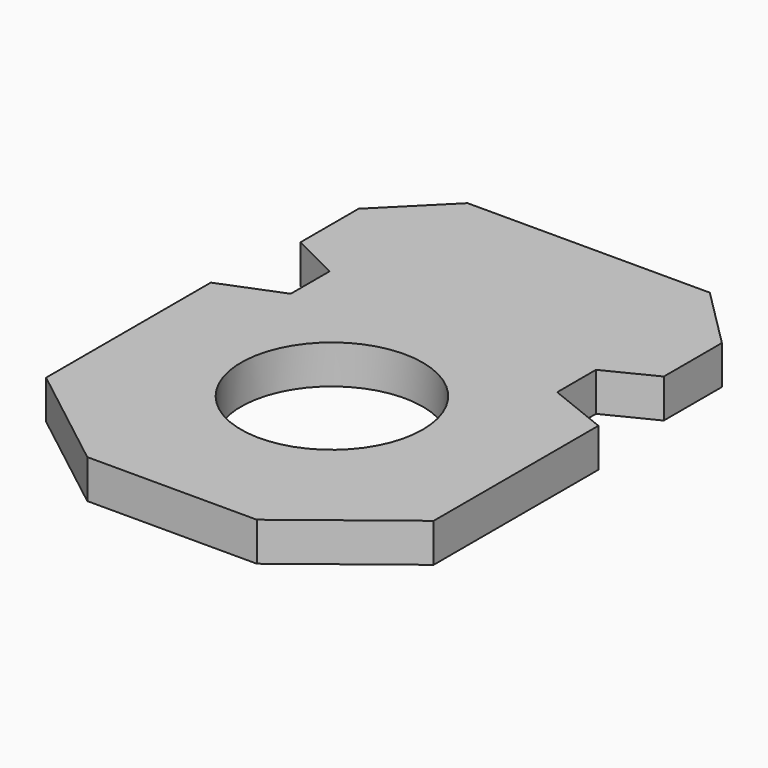
from build123d import *

# Parameters (mm, degrees)
F0_R     = 7.5
F1_DEPTH = 3.2
F2_SIZE2 = 7
F2_SIZE  = 9
F3_SIZE  = 5


with BuildPart() as f1:
    # F0 (on Top) → F1 (new body)
    with BuildSketch(Plane.XY):
        Polygon((-16, 0), (-16, -24), (16, -24), (16, 0), (11, 2), (11, 6), (15, 8), (15, 19), (-15, 19), (-15, 8), (-11, 6), (-11, 2), align=None)
        with Locations((0, -7.5)):
            Circle(F0_R, mode=Mode.SUBTRACT)
    extrude(amount=F1_DEPTH)

    # F2
    f2_edges = [f1.edges().sort_by_distance(p)[0] for p in [
        (-16, -24, 1.6),
        (16, -24, 1.6),
    ]]
    f2_side = f1.faces().sort_by_distance((0, -24, 1.6))[0]
    chamfer(f2_edges, length=F2_SIZE, length2=F2_SIZE2, reference=f2_side)

    # F3
    f3_edges = [f1.edges().sort_by_distance(p)[0] for p in [
        (-15, 19, 1.6),
        (15, 19, 1.6),
    ]]
    chamfer(f3_edges, length=F3_SIZE)


solid = f1.part
